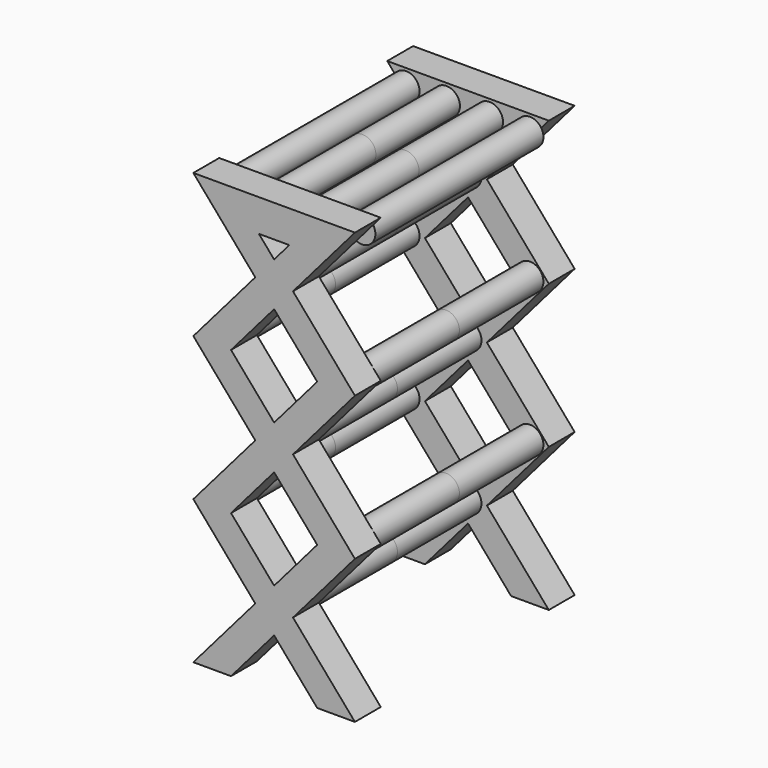
from build123d import *

# Parameters (mm, degrees)
F1_DEPTH = 76.2
F2_R     = 31.75
F3_DEPTH = 247.65


# Not quite as in the source:
# - a feature names something its author has since deleted; it is built from what else it names


with BuildPart() as f1:
    # F0 (on Front) → F1 (new body)
    with BuildSketch(Plane.XZ):
        Polygon((-234.95, 507.873), (-190.5, 559.3963478261), (-292.1, 677.164), (-381, 677.164), align=None)
        Polygon((-190.5, 456.3496521739), (-146.05, 507.873), (-190.5, 559.3963478261), (-234.95, 507.873), align=None)
        Polygon((-190.5, 559.3963478261), (-146.05, 507.873), (0, 677.164), (-88.9, 677.164), align=None)
        Polygon((-88.9, 338.582), (0, 338.582), (-146.05, 507.873), (-190.5, 456.3496521739), align=None)
        Polygon((-381, 338.582), (-292.1, 338.582), (-190.5, 456.3496521739), (-234.95, 507.873), align=None)
        Polygon((-234.95, 169.291), (-190.5, 220.8143478261), (-292.1, 338.582), (-381, 338.582), align=None)
        Polygon((-190.5, 220.8143478261), (-146.05, 169.291), (0, 338.582), (-88.9, 338.582), align=None)
        Polygon((-190.5, 117.7676521739), (-146.05, 169.291), (-190.5, 220.8143478261), (-234.95, 169.291), align=None)
        Polygon((-88.9, 0), (0, 0), (-146.05, 169.291), (-190.5, 117.7676521739), align=None)
        Polygon((-292.1, 0), (-190.5, 117.7676521739), (-234.95, 169.291), (-381, 0), align=None)
        Polygon((-381, 677.164), (-292.1, 677.164), (-190.5, 794.9316521739), (-234.95, 846.455), align=None)
        Polygon((-190.5, 794.9316521739), (-146.05, 846.455), (-190.5, 897.9783478261), (-234.95, 846.455), align=None)
        Polygon((-88.9, 677.164), (0, 677.164), (-146.05, 846.455), (-190.5, 794.9316521739), align=None)
        Polygon((-190.5, 897.9783478261), (-146.05, 846.455), (0, 1015.746), (-88.9, 1015.746), (-154.6389347337, 939.546), align=None)
        Polygon((-154.6389347337, 939.546), (-88.9, 1015.746), (-292.1, 1015.746), (-226.3610652663, 939.546), align=None)
        Polygon((-234.95, 846.455), (-190.5, 897.9783478261), (-226.3610652663, 939.546), (-292.1, 1015.746), (-381, 1015.746), align=None)
    extrude(amount=F1_DEPTH)

    # F2 (on face) → F3 (join)
    with BuildSketch(Plane.XZ.offset(76.2)):
        with Locations((-336.55, 677.164)):
            Circle(F2_R)
        with Locations((-44.45, 677.164)):
            Circle(F2_R)
        with Locations((-190.5, 507.873)):
            Circle(F2_R)
        with Locations((-190.5, 169.291)):
            Circle(F2_R)
        with Locations((-44.45, 338.582)):
            Circle(F2_R)
        with Locations((-336.55, 338.582)):
            Circle(F2_R)
        with Locations((-190.5, 846.455)):
            Circle(F2_R)
        with Locations((-44.45, 977.646)):
            Circle(F2_R)
        with Locations((-139.7, 977.646)):
            Circle(F2_R)
        with Locations((-336.55, 977.646)):
            Circle(F2_R)
        with Locations((-241.3, 977.646)):
            Circle(F2_R)
    extrude(amount=F3_DEPTH)

    # F4: F1 across face


with BuildPart() as f1_1:
    add(f1.part)
    add(f1.part.mirror(Plane(origin=(-336.55, -323.85, 977.646), x_dir=(1, 0, 0), z_dir=(0, -1, 0))))


solid = f1_1.part
